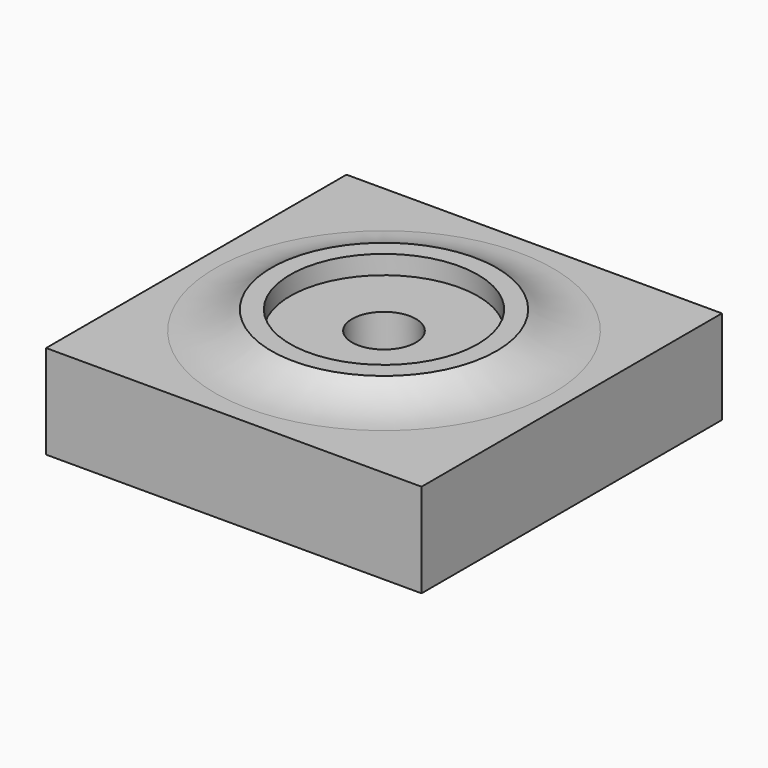
from build123d import *

# Parameters (mm, degrees)
F0_W           = 20
F0_H           = 20
F0_R           = 6
F0_R_2         = 5
F0_R_3         = 3.5
F1_DEPTH       = 5
F2_DEPTH       = 6
F3_DEPTH       = 1
F4_D           = 3.4
F4_START       = 1
F4_CSINK_D     = 6.72
F4_CSINK_ANGLE = 90
F6_ANGLE       = 180


# Not quite as in the source:
# - a fillet or chamfer that OpenCascade refuses, or shapes differently, is made with other operations: its cross-section is extruded or revolved along the edge and cut away or added


with BuildPart() as f1:
    # F0 (on Top) → F1 (new body)
    with BuildSketch(Plane.XY):
        Rectangle(F0_W, F0_H)
        Circle(F0_R, mode=Mode.SUBTRACT)
        Circle(F0_R)
        Circle(F0_R_2, mode=Mode.SUBTRACT)
        Circle(F0_R_2)
        Circle(F0_R_3, mode=Mode.SUBTRACT)
        Circle(F0_R_3)
    extrude(amount=-F1_DEPTH)

    # F0 (on Top) → F2 (join)
    with BuildSketch(Plane.XY):
        Circle(F0_R)
        Circle(F0_R_2, mode=Mode.SUBTRACT)
    extrude(amount=-F2_DEPTH)

    # F0 (on Top) → F3 (cut)
    with BuildSketch(Plane.XY):
        Circle(F0_R_3)
    extrude(amount=-F3_DEPTH, mode=Mode.SUBTRACT)

    # F4 (through all)
    # its depths count from where the whole tool has entered the part; down to there all is cleared
    with Locations(Plane.XY.offset(-F4_START)):
        with Locations((0, 0)):
            CounterSinkHole(F4_D / 2, F4_CSINK_D / 2, counter_sink_angle=F4_CSINK_ANGLE)

    # F5: fillet of radius 5 on 1 edges, made by hand

    # F5_s1 → F5_t2 (revolve)
    with BuildSketch(Plane.XZ):
        with BuildLine():
            ThreePointArc((9, -5), (7.4188611699, -5.2565835097), (6, -6))
            Line((6, -6), (5.94, -5.92))
            ThreePointArc((5.94, -5.92), (5.9, -5.5), (5.9, -5))
            Line((5.9, -5), (6, -4.9))
            Line((6, -4.9), (9, -4.9))
            Line((9, -4.9), (9, -5))
        make_face()
    revolve(axis=Axis((0, 0, -5), (0, 0, 1)))


with BuildPart() as f1_1:
    # F6: moved
    add(f1.part.rotate(Axis((0, 10, 0), (-1, 0, 0)), F6_ANGLE))


solid = f1_1.part
